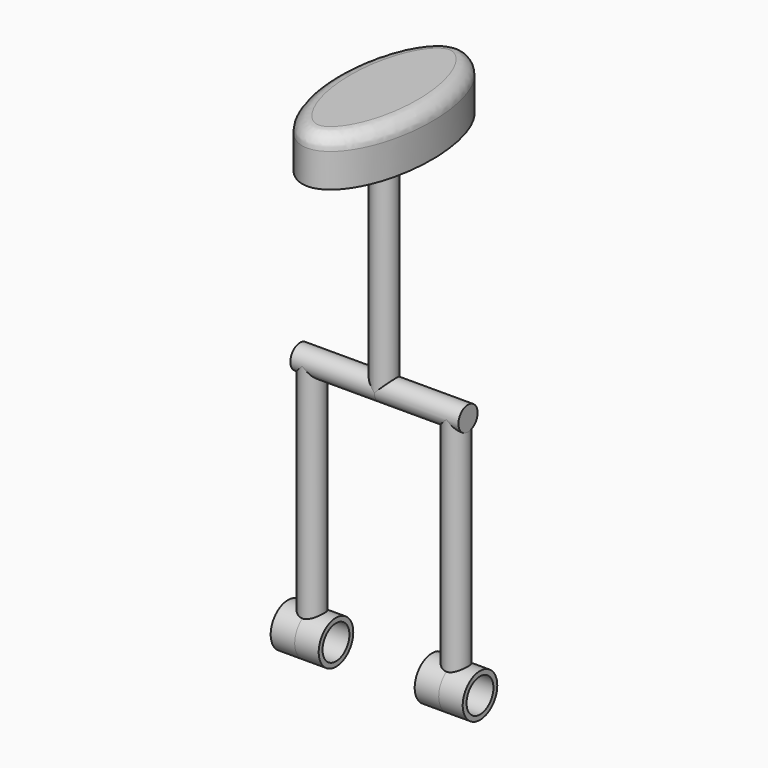
from build123d import *
from build123d import SkipClean  # not in build123d's __all__

# Parameters (mm, degrees)
F1_DEPTH       = 10
F2_R           = 2.5
F3_DEPTH       = 45
F4_R           = 2.5
F5_DEPTH       = 17.5
F5_DEPTH_BACK  = 17.5
F7_R           = 2.5
F8_DEPTH       = 50
F12_R          = 4.5
F13_DEPTH      = 5
F13_DEPTH_BACK = 5
F14_R          = 3.5
F15_DEPTH      = 25
F16_R          = 4.5
F17_DEPTH      = 5
F17_DEPTH_BACK = 5
F18_R          = 3.5
F19_DEPTH      = 25
F20_R          = 3


with BuildPart() as f1:
    # F0 (on Top) → F1 (new body)
    with BuildSketch(Plane.XY):
        with BuildLine():
            add(Edge.make_bspline(
                [(0, 20), (-17.3205080757, 20), (-8.6602540378, -10), (0, -40), (8.6602540378, -10), (17.3205080757, 20), (0, 20)],
                knots=[0, 0, 0, 2.0943951024, 2.0943951024, 4.1887902048, 4.1887902048, 6.2831853072, 6.2831853072, 6.2831853072], degree=2, weights=[1, 0.5, 1, 0.5, 1, 0.5, 1]))
        make_face()
    extrude(amount=F1_DEPTH)

    # F2 (on face) → F3 (join)
    with BuildSketch(Plane(origin=(0, 0, 0), x_dir=(1, 0, 0), z_dir=(0, 0, -1))):
        Circle(F2_R)
    extrude(amount=F3_DEPTH)

    # F4 (on Right) → F5 (join, two sides)
    with BuildSketch(Plane.YZ) as f5_sk:
        with Locations((0, -45)):
            Circle(F4_R)
    extrude(amount=F5_DEPTH)
    extrude(f5_sk.sketch, amount=-F5_DEPTH_BACK)

    # F7 (on offset) → F8 (join)
    with BuildSketch(Plane.XY.offset(-45)):
        with Locations((15, 0)):
            Circle(F7_R)
        with Locations((-15, 0)):
            Circle(F7_R)
    with SkipClean():  # cleaning this boolean's faces spoils the solid; the shape is the same uncleaned
        extrude(amount=-F8_DEPTH)


with BuildPart() as f1_1:
    # F9: moved
    add(f1.part.moved(Location((0, 0, 45))), clean=False)

    # F12 (on offset) → F13 (join, two sides)
    with BuildSketch(Plane.YZ.offset(15)) as f13_sk:
        with Locations((0, -50)):
            Circle(F12_R)
    extrude(amount=F13_DEPTH)
    extrude(f13_sk.sketch, amount=-F13_DEPTH_BACK)

    # F14 (on face) → F15 (cut)
    with BuildSketch(Plane.YZ.offset(20)):
        with Locations((0, -50)):
            Circle(F14_R)
    extrude(amount=-F15_DEPTH, mode=Mode.SUBTRACT)

    # F16 (on offset) → F17 (join, two sides)
    with BuildSketch(Plane.YZ.offset(-15)) as f17_sk:
        with Locations((0, -50)):
            Circle(F16_R)
    extrude(amount=F17_DEPTH)
    extrude(f17_sk.sketch, amount=-F17_DEPTH_BACK)

    # F18 (on face) → F19 (cut)
    with BuildSketch(Plane(origin=(-20, 0, 0), x_dir=(0, -1, 0), z_dir=(-1, 0, 0))):
        with Locations((0, -50)):
            Circle(F18_R)
    extrude(amount=-F19_DEPTH, mode=Mode.SUBTRACT)

    # F20
    f20_edges = [f1_1.edges().sort_by_distance(p)[0] for p in [
        (-2e-06, -20, 55),
    ]]
    fillet(f20_edges, radius=F20_R)


solid = f1_1.part
